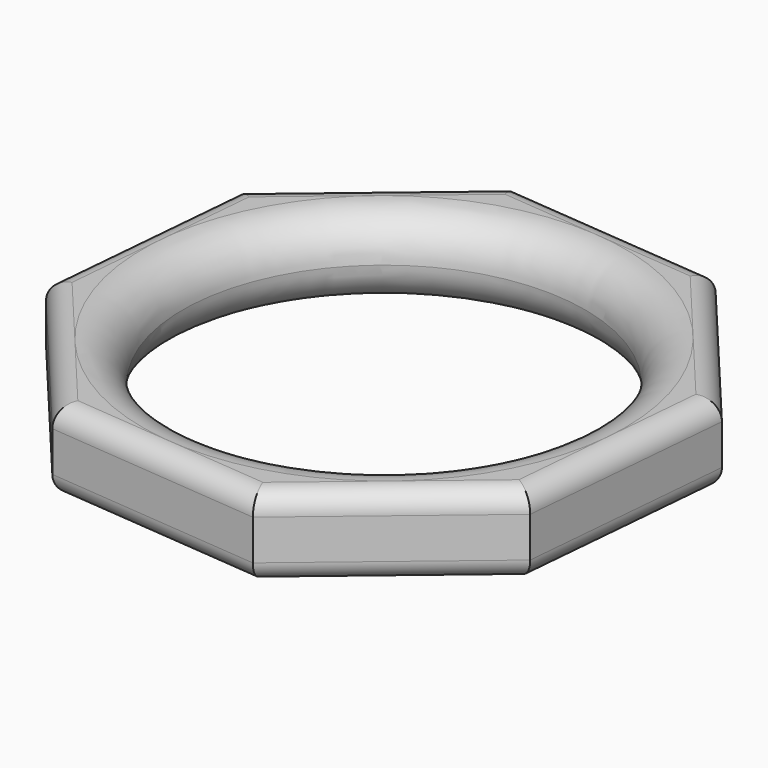
from build123d import *

# Parameters (mm, degrees)
F0_R     = 10
F1_DEPTH = 4
F2_R     = 1.99999
F3_R     = 1


# Not quite as in the source:
# - a fillet or chamfer is up to 0.001 mm smaller than in the source, because OpenCascade refuses the exact size


with BuildPart() as f1:
    # F0 (on Top) → F1 (new body)
    with BuildSketch(Plane.XY):
        Polygon((4.2186513593, -13.4238145334), (12.4751072696, -6.5090333023), (13.4238145334, 4.2186513593), (6.5090333023, 12.4751072696), (-4.2186513593, 13.4238145334), (-12.4751072696, 6.5090333023), (-13.4238145334, -4.2186513593), (-6.5090333023, -12.4751072696), align=None)
        Circle(F0_R, mode=Mode.SUBTRACT)
    extrude(amount=F1_DEPTH)

    # F2 (radius 2 in the source; OpenCascade refuses exactly that, so slightly less here)
    f2_edges = [f1.edges().sort_by_distance(p)[0] for p in [
        (-10, 0, 0),
        (-10, 0, 4),
    ]]
    fillet(f2_edges, radius=F2_R)

    # F3
    f3_edges = [f1.edges().sort_by_distance(p)[0] for p in [
        (1.145191, 12.949461, 4),
        (-8.346879, 9.966424, 4),
        (-12.949461, 1.145191, 4),
        (-9.966424, -8.346879, 4),
        (-1.145191, -12.949461, 4),
        (8.346879, -9.966424, 4),
        (12.949461, -1.145191, 4),
        (9.966424, 8.346879, 4),
        (9.966424, 8.346879, 0),
        (12.949461, -1.145191, 0),
        (8.346879, -9.966424, 0),
        (-1.145191, -12.949461, 0),
        (-9.966424, -8.346879, 0),
        (-12.949461, 1.145191, 0),
        (-8.346879, 9.966424, 0),
        (1.145191, 12.949461, 0),
    ]]
    fillet(f3_edges, radius=F3_R)


solid = f1.part
